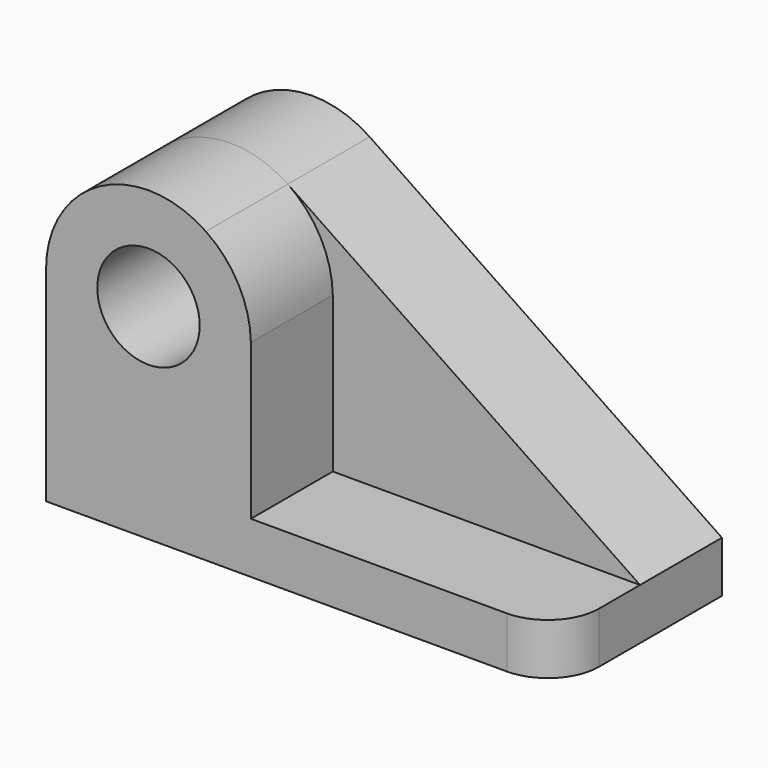
from build123d import *

# Parameters (mm, degrees)
F0_R     = 12.7
F1_DEPTH = 25.4
F2_R     = 12.7
F3_DEPTH = 25.4
F4_R     = 12.7


# Not quite as in the source:
# - ends of sketch curves that miss each other by under 0.0002 mm in the source are joined


with BuildPart() as f1:
    # F0 (on Front) → F1 (new body)
    with BuildSketch(Plane.XZ):
        with BuildLine():
            Line((50.5598429927, -25.9062238405), (-36.8059224535, 33.2085917174))
            ThreePointArc((-36.8059224535, 33.2085917174), (-62.9386576581, 34.612527229), (-76.4401570073, 12.1937761595))
            ThreePointArc((-76.4401570073, 12.1937761595), (-76.4401641327, 12.1827917596), (-76.4401665079, 12.1718073576))
            Line((-76.4401665079, 12.1718073576), (-76.4401570073, -38.6062238405))
            Line((-76.4401570073, -38.6062238405), (50.5598429927, -38.6062238405))
            Line((50.5598429927, -38.6062238405), (50.5598429927, -25.9062238405))
        make_face()
        with Locations((-51.0401665079, 12.1718073576)):
            Circle(F0_R, mode=Mode.SUBTRACT)
    extrude(amount=F1_DEPTH)

    # F2 (on face) → F3 (join)
    with BuildSketch(Plane.XZ.offset(25.4)):
        with BuildLine():
            Line((-25.643836125, -25.9062238405), (-25.643836125, 11.740622413))
            Line((-25.643836125, 11.740622413), (-25.643836125, 12.6029923022))
            ThreePointArc((-25.643836125, 12.6029923022), (-28.7064900796, 24.2700061726), (-36.8059277776, 33.2085838488))
            ThreePointArc((-36.8059277776, 33.2085838488), (-62.9386532076, 34.6125188354), (-76.4401475068, 12.1937761513))
            ThreePointArc((-76.4401475068, 12.1937761513), (-76.4401546322, 12.1827917555), (-76.4401570073, 12.1718073576))
            Line((-76.4401570073, 12.1718073576), (-76.4401570073, -25.9062238405))
            Line((-76.4401570073, -25.9062238405), (-76.4401570073, -38.6062238405))
            Line((-76.4401570073, -38.6062238405), (50.5598429927, -38.6062238405))
            Line((50.5598429927, -38.6062238405), (50.5598429927, -25.9062238405))
            Line((50.5598429927, -25.9062238405), (-25.643836125, -25.9062238405))
        make_face()
        with Locations((-51.0401665079, 12.1718073576)):
            Circle(F2_R, mode=Mode.SUBTRACT)
    extrude(amount=F3_DEPTH)

    # F4
    f4_edges = [f1.edges().sort_by_distance(p)[0] for p in [
        (50.559843, -50.8, -32.256224),
    ]]
    fillet(f4_edges, radius=F4_R)


solid = f1.part
